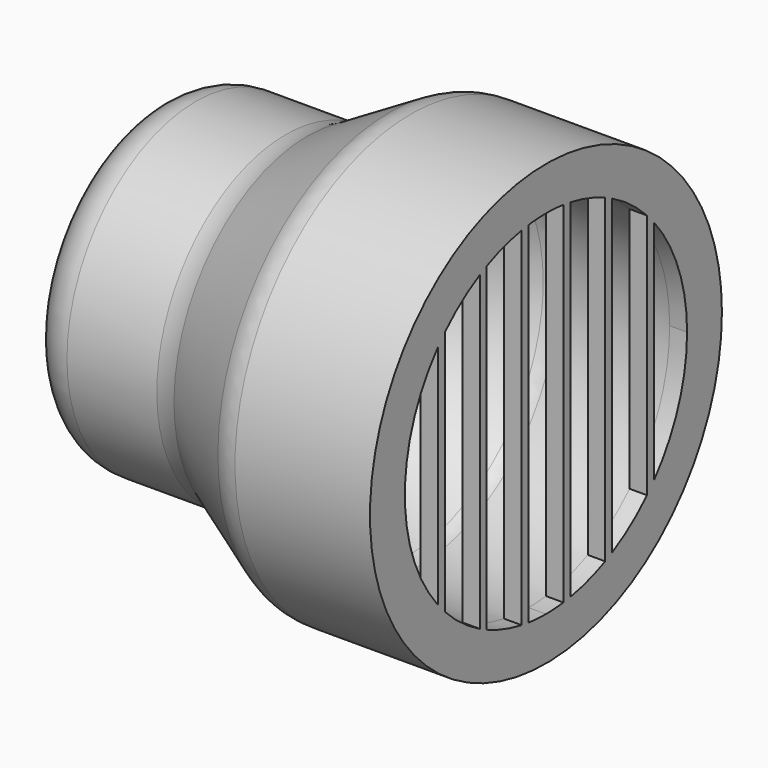
from build123d import *

# Parameters (mm, degrees)
F2_R     = 25.25
F3_DEPTH = 2
F5_DEPTH = 2
F6_R     = 4.99999
F7_R     = 3


# Not quite as in the source:
# - a fillet or chamfer is up to 0.001 mm smaller than in the source, because OpenCascade refuses the exact size
# - a feature names something its author has since deleted; it is built from what else it names


with BuildPart() as f1:
    # F0 (on Top) → F1 (revolve)
    with BuildSketch(Plane.XY):
        Polygon((-18, 18.5), (-18, 13.5), (0, 13.5), (11.6913429511, 20.25), (25.1913429511, 20.25), (25.1913429511, 25.25), (10.3515969889, 25.25), (-1.3397459622, 18.5), align=None)
    revolve(axis=Axis((-8.7595172226, 0, 0), (1, 0, 0)))

    # F2 (on face) → F3 (join)
    with BuildSketch(Plane.YZ.offset(25.1913429511)):
        Circle(F2_R)
    extrude(amount=F3_DEPTH)

    # F4 (on face) → F5 (cut, through all)
    with BuildSketch(Plane.YZ.offset(27.1913429511)):
        with BuildLine():
            ThreePointArc((14.5, 14.1355049432), (12.1454310832, 16.2034256811), (9.5, 17.8833022678))
            Line((9.5, 17.8833022678), (9.5, -17.8833022678))
            ThreePointArc((9.5, -17.8833022678), (12.1454310832, -16.2034256811), (14.5, -14.1355049432))
            Line((14.5, -14.1355049432), (14.5, 14.1355049432))
        make_face()
        with BuildLine():
            ThreePointArc((8.5, 18.3796762757), (6.0508466769, 19.3248481105), (3.5, 19.9452375268))
            Line((3.5, 19.9452375268), (3.5, -19.9452375268))
            ThreePointArc((3.5, -19.9452375268), (6.0508466769, -19.3248481105), (8.5, -18.3796762757))
            Line((8.5, -18.3796762757), (8.5, 18.3796762757))
        make_face()
        with BuildLine():
            ThreePointArc((2.5, 20.0950864641), (1.2523975211, 20.2112345108), (0, 20.25))
            ThreePointArc((0, 20.25), (-1.2523975211, 20.2112345108), (-2.5, 20.0950864641))
            Line((-2.5, 20.0950864641), (-2.5, -20.0950864641))
            ThreePointArc((-2.5, -20.0950864641), (-1.2523975211, -20.2112345108), (0, -20.25))
            ThreePointArc((0, -20.25), (1.2523975211, -20.2112345108), (2.5, -20.0950864641))
            Line((2.5, -20.0950864641), (2.5, 20.0950864641))
        make_face()
        with BuildLine():
            Line((-3.5, -19.9452375268), (-3.5, 19.9452375268))
            ThreePointArc((-3.5, 19.9452375268), (-6.0508466769, 19.3248481105), (-8.5, 18.3796762757))
            Line((-8.5, 18.3796762757), (-8.5, -18.3796762757))
            ThreePointArc((-8.5, -18.3796762757), (-6.0508466769, -19.3248481105), (-3.5, -19.9452375268))
        make_face()
        with BuildLine():
            Line((-9.5, -17.8833022678), (-9.5, 17.8833022678))
            ThreePointArc((-9.5, 17.8833022678), (-12.1454310832, 16.2034256811), (-14.5, 14.1355049432))
            Line((-14.5, 14.1355049432), (-14.5, -14.1355049432))
            ThreePointArc((-14.5, -14.1355049432), (-12.1454310832, -16.2034256811), (-9.5, -17.8833022678))
        make_face()
        with BuildLine():
            Line((-15.5, -13.0312125299), (-15.5, 13.0312125299))
            ThreePointArc((-15.5, 13.0312125299), (-20.25, 0), (-15.5, -13.0312125299))
        make_face()
        with BuildLine():
            ThreePointArc((20.25, 0), (19.0254763409, 6.9349657533), (15.5, 13.0312125299))
            Line((15.5, 13.0312125299), (15.5, -13.0312125299))
            ThreePointArc((15.5, -13.0312125299), (19.0254763409, -6.9349657533), (20.25, 0))
        make_face()
    extrude(amount=-F5_DEPTH, mode=Mode.SUBTRACT)

    # F6 (radius 5 in the source; OpenCascade refuses exactly that, so slightly less here)
    f6_edges = [f1.edges().sort_by_distance(p)[0] for p in [
        (-18, -18.5, 0),
        (-1.339746, -18.5, 0),
        (10.351597, -25.25, 0),
    ]]
    fillet(f6_edges, radius=F6_R)

    # F7
    f7_edges = [f1.edges().sort_by_distance(p)[0] for p in [
        (11.691343, -20.25, 0),
        (0, -13.5, 0),
    ]]
    fillet(f7_edges, radius=F7_R)


solid = f1.part
